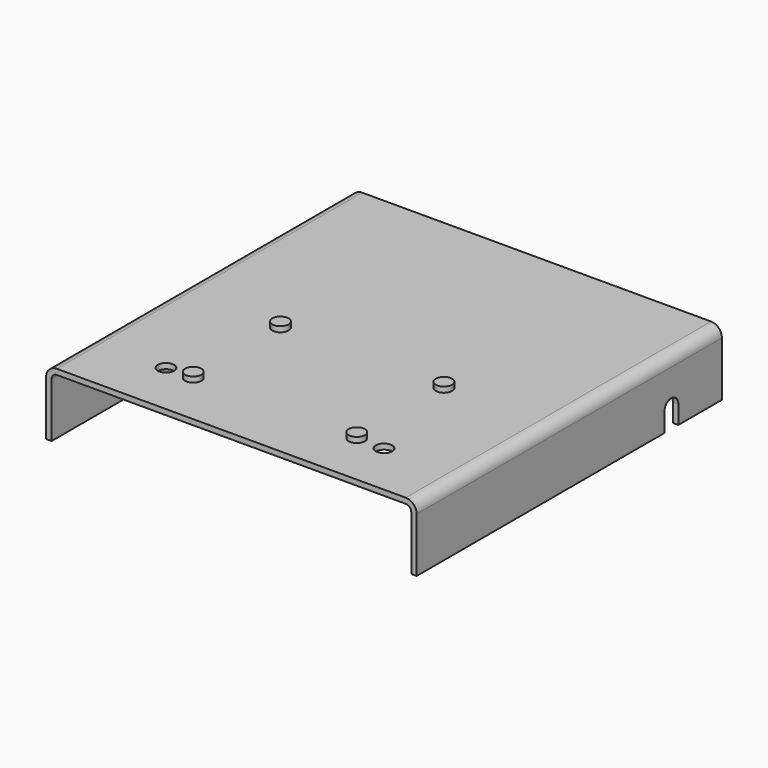
from build123d import *

# Parameters (mm, degrees)
F1_DEPTH = 350
F3_DEPTH = 340.0010036672
F4_R     = 7.5
F5_DEPTH = 5
F6_R     = 7.5
F7_DEPTH = 5


# Not quite as in the source:
# - ends of sketch curves that miss each other by under 0.0002 mm in the source are joined


with BuildPart() as f1:
    # F0 (on Front) → F1 (new body)
    with BuildSketch(Plane.XZ):
        with BuildLine():
            Line((160, -88.7002011906), (-160.0000036672, -88.7002011906))
            ThreePointArc((-160.0000036672, -88.7002011906), (-167.0710714791, -91.6291333788), (-170.0000036672, -98.7002011906))
            Line((-170.0000036672, -98.7002011906), (-170, -148.7002011906))
            Line((-170, -148.7002011906), (-165.0000036672, -148.7002011906))
            Line((-165.0000036672, -148.7002011906), (-165.0000036672, -98.7002011906))
            ThreePointArc((-165.0000036672, -98.7002011906), (-163.5355375731, -95.1646672847), (-160.0000036672, -93.7002011906))
            Line((-160.0000036672, -93.7002011906), (160, -93.7002011906))
            ThreePointArc((160, -93.7002011906), (163.5355339059, -95.1646672847), (165, -98.7002011906))
            Line((165, -98.7002011906), (165, -148.7002011906))
            Line((165, -148.7002011906), (170, -148.7002011906))
            Line((170, -148.7002011906), (170, -98.7002011906))
            ThreePointArc((170, -98.7002011906), (167.0710678119, -91.6291333788), (160, -88.7002011906))
        make_face()
    extrude(amount=F1_DEPTH)

    # F2 (on face) → F3 (cut, through all)
    with BuildSketch(Plane.YZ.offset(170)):
        with BuildLine():
            Line((-66, -148.7002011906), (-50, -148.7002011906))
            Line((-50, -148.7002011906), (-50, -131.7002011906))
            ThreePointArc((-50, -131.7002011906), (-52.3431457505, -126.0433469411), (-58, -123.7002011906))
            ThreePointArc((-58, -123.7002011906), (-63.6568542495, -126.0433469411), (-66, -131.7002011906))
            Line((-66, -131.7002011906), (-66, -148.7002011906))
        make_face()
    extrude(amount=-F3_DEPTH, mode=Mode.SUBTRACT)

    # F4 (on face) → F5 (cut, through all)
    with BuildSketch(Plane.XY.offset(-88.7002011906)):
        with Locations((-100, -300)):
            Circle(F4_R)
        with Locations((100, -300)):
            Circle(F4_R)
    extrude(amount=-F5_DEPTH, mode=Mode.SUBTRACT)

    # F6 (on face) → F7 (join)
    with BuildSketch(Plane.XY.offset(-88.7002011906)):
        with Locations((-75, -200)):
            Circle(F6_R)
        with Locations((-75, -300)):
            Circle(F6_R)
        with Locations((75, -300)):
            Circle(F6_R)
        with Locations((75, -200)):
            Circle(F6_R)
    extrude(amount=F7_DEPTH)


solid = f1.part
